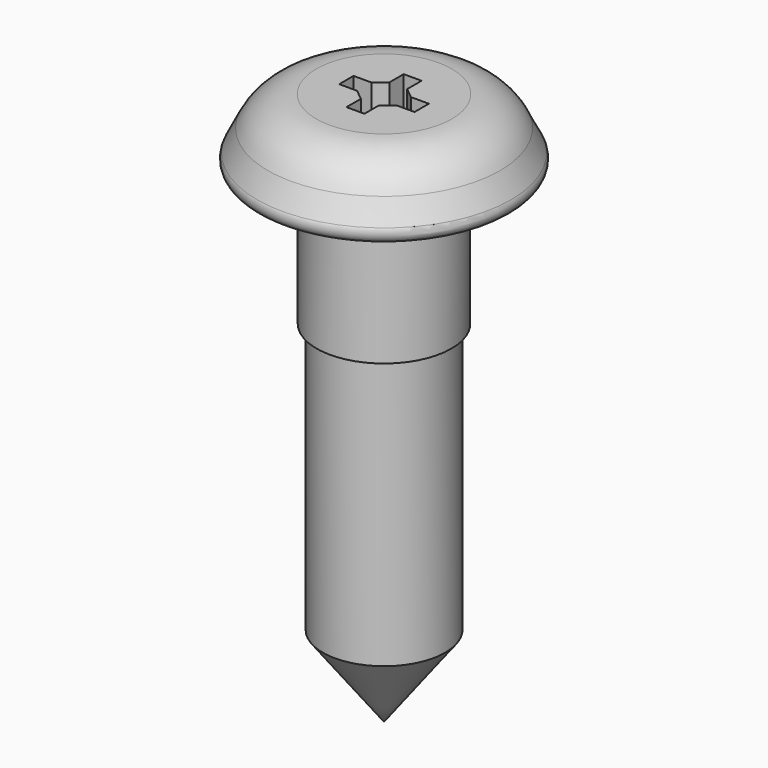
from build123d import *

# Parameters (mm, degrees)
F0_R      = 3.175
F2_R      = 2.38125
F4_R      = 1.27
F5_R      = 0.254
F7_DEPTH  = 1.5875
F8_R      = 1.5875
F9_DEPTH  = 3.175
F10_R     = 1.4422766601
F11_DEPTH = 6.35


# Not quite as in the source:
# - a length typed as a fraction of an inch, garbled in the dataset ("3 / 203.2 mm" for 3/8 in), is restored


with BuildPart() as f3:
    # F0 (on Top) → F3 section 0
    with BuildSketch(Plane.XY):
        Circle(F0_R)
    # F2 (on offset) → F3 section 1
    with BuildSketch(Plane.XY.offset(1.5875)):
        Circle(F2_R)
    loft()

    # F4
    f4_edges = [f3.edges().sort_by_distance(p)[0] for p in [
        (-2.38125, 0, 1.5875),
    ]]
    fillet(f4_edges, radius=F4_R)

    # F5
    f5_edges = [f3.edges().sort_by_distance(p)[0] for p in [
        (-3.175, 0, 0),
    ]]
    fillet(f5_edges, radius=F5_R)

    # F6 (on face) → F7 (cut)
    with BuildSketch(Plane.XY.offset(1.5875)):
        Polygon((-0.2111591544, 0.8412458697), (-0.2111591544, 0.4189275609), (-0.4643816895, 0.2111591544), (-0.8866999983, 0.2111591544), (-0.8866999983, -0.2111591544), (-0.4643816895, -0.2111591544), (-0.2111591544, -0.4189275609), (-0.2111591544, -0.8412458697), (0.2111591544, -0.8412458697), (0.2111591544, -0.4189275609), (0.4643816895, -0.2111591544), (0.8866999983, -0.2111591544), (0.8866999983, 0.2111591544), (0.4643816895, 0.2111591544), (0.2111591544, 0.4189275609), (0.2111591544, 0.8412458697), align=None)
    extrude(amount=-F7_DEPTH, mode=Mode.SUBTRACT)

    # F8 (on Top) → F9 (join)
    with BuildSketch(Plane.XY):
        Circle(F8_R)
    extrude(amount=-F9_DEPTH)

    # F10 (on face) → F11 (join)
    with BuildSketch(Plane(origin=(0, 0, -3.175), x_dir=(1, 0, 0), z_dir=(0, 0, -1))):
        Circle(F10_R)
    extrude(amount=F11_DEPTH)

    # F12 (on Right) → F13 (revolve)
    with BuildSketch(Plane.YZ):
        Polygon((0, -11.43), (1.4422766601, -9.525), (0, -9.525), align=None)
    revolve(axis=Axis((0, 0, -10.4775), (0, 0, 1)))


solid = f3.part
